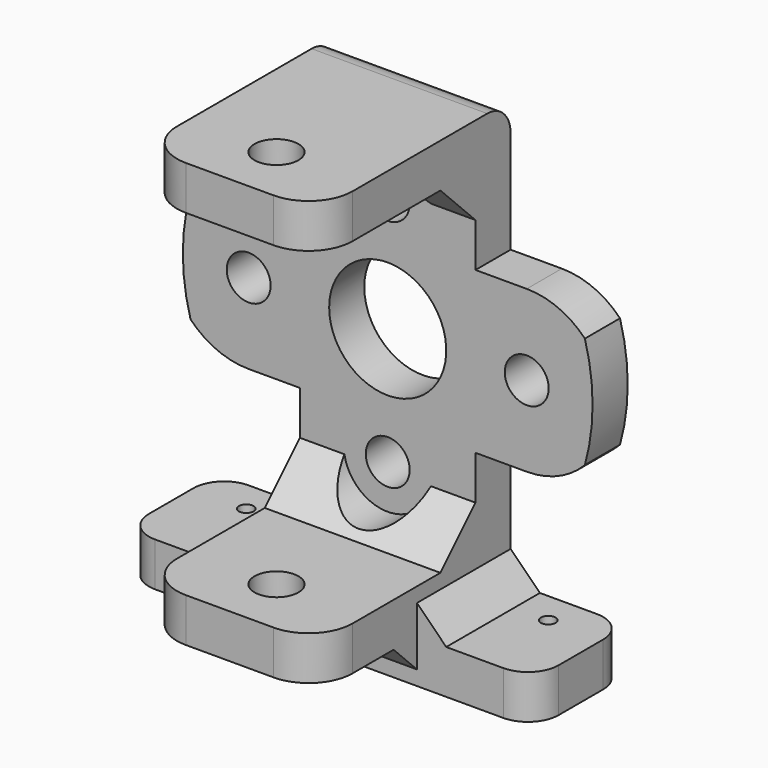
from build123d import *

# Parameters (mm, degrees)
F0_R          = 1.5
F0_R_2        = 4.5
F1_DEPTH      = 3
F2_W          = 12
F2_H          = 29
F3_DEPTH      = 3
F4_R          = 1.5
F5_DEPTH      = 3
F6_R          = 4
F6_R_2        = 1.5
F7_DEPTH      = 3
F9_R          = 2
F10_T4_DEPTH  = 12
F10_S5_R      = 1.5
F10_T6_DEPTH  = 8
F10_T10_DEPTH = 12
F10_S11_R     = 1.5
F10_T12_DEPTH = 8
F11_R         = 3
F12_DEPTH     = 4
F13_R         = 0.5
F14_DEPTH     = 3
F15_T1_DEPTH  = 8
F16_T1_DEPTH  = 8
F17_SIZE      = 2


# Not quite as in the source:
# - a fillet or chamfer that OpenCascade refuses, or shapes differently, is made with other operations: its cross-section is extruded or revolved along the edge and cut away or added


with BuildPart() as f1:
    # F0 (on Front) → F1 (new body)
    with BuildSketch(Plane.XZ):
        with BuildLine():
            Line((0, -5.5), (9.5, -5.5))
            ThreePointArc((9.5, -5.5), (11.6605151609, -5.0578823869), (13.4736842105, -3.8026088144))
            ThreePointArc((13.4736842105, -3.8026088144), (14, 0), (13.4736842105, 3.8026088144))
            ThreePointArc((13.4736842105, 3.8026088144), (11.6605151609, 5.0578823869), (9.5, 5.5))
            Line((9.5, 5.5), (0, 5.5))
            Line((0, 5.5), (-9.5, 5.5))
            ThreePointArc((-9.5, 5.5), (-11.6605151609, 5.0578823869), (-13.4736842105, 3.8026088144))
            ThreePointArc((-13.4736842105, 3.8026088144), (-14, 0), (-13.4736842105, -3.8026088144))
            ThreePointArc((-13.4736842105, -3.8026088144), (-11.6605151609, -5.0578823869), (-9.5, -5.5))
            Line((-9.5, -5.5), (0, -5.5))
        make_face()
        with Locations((-9.5, 0)):
            Circle(F0_R, mode=Mode.SUBTRACT)
        Circle(F0_R_2, mode=Mode.SUBTRACT)
        with Locations((9.5, 0)):
            Circle(F0_R, mode=Mode.SUBTRACT)
    extrude(amount=F1_DEPTH)

    # F2 (on face) → F3 (join)
    with BuildSketch(Plane.XZ.offset(3)):
        Rectangle(F2_W, F2_H)
    extrude(amount=-F3_DEPTH)

    # F4 (on face) → F5 (join)
    with BuildSketch(Plane(origin=(0, 0, -14.5), x_dir=(1, 0, 0), z_dir=(0, 0, -1))):
        with BuildLine():
            Line((-6, 13.5), (-6, 0))
            Line((-6, 0), (6, 0))
            Line((6, 0), (6, 13.5))
            ThreePointArc((6, 13.5), (5.1213203436, 15.6213203436), (3, 16.5))
            Line((3, 16.5), (-3, 16.5))
            ThreePointArc((-3, 16.5), (-5.1213203436, 15.6213203436), (-6, 13.5))
        make_face()
        with Locations((0, 12.5)):
            Circle(F4_R, mode=Mode.SUBTRACT)
    extrude(amount=-F5_DEPTH)

    # F6 (on face) → F7 (cut, through all)
    with BuildSketch(Plane(origin=(0, 0, 0), x_dir=(-1, 0, 0), z_dir=(0, 1, 0))):
        Circle(F6_R)
        with Locations((0, 8)):
            Circle(F6_R_2)
        with Locations((0, -8)):
            Circle(F6_R_2)
    extrude(amount=-F7_DEPTH, mode=Mode.SUBTRACT)

    # F8: F1 across plane


with BuildPart() as f1_1:
    add(f1.part)
    add(f1.part.mirror(Plane.XY))

    # F9
    f9_edges = [f1_1.edges().sort_by_distance(p)[0] for p in [
        (0, 0, 14.5),
    ]]
    fillet(f9_edges, radius=F9_R)

    # F10: chamfer of 3 on 2 edges, made by hand


with BuildPart() as f10_tool2:
    # F10_s3 → F10_t4 (new body)
    with BuildSketch(Plane.YZ.offset(-6)):
        Polygon((-3, 8.5), (-6, 11.5), (-3, 11.5), align=None)
    extrude(amount=F10_T4_DEPTH)

    # F10_s5 → F10_t6 (cut, symmetric)
    with BuildSketch(Plane.XZ.offset(4.5)):
        with Locations((0, 8)):
            Circle(F10_S5_R)
    extrude(amount=F10_T6_DEPTH, both=True, mode=Mode.SUBTRACT)


with BuildPart() as f1_2:
    add(f1_1.part)

    # F10_t1: union F10_tool2
    add(f10_tool2.part)


with BuildPart() as f10_tool8:
    # F10_s9 → F10_t10 (new body)
    with BuildSketch(Plane.YZ.offset(-6)):
        Polygon((-3, -8.5), (-6, -11.5), (-3, -11.5), align=None)
    extrude(amount=F10_T10_DEPTH)

    # F10_s11 → F10_t12 (cut, symmetric)
    with BuildSketch(Plane.XZ.offset(4.5)):
        with Locations((0, -8)):
            Circle(F10_S11_R)
    extrude(amount=F10_T12_DEPTH, both=True, mode=Mode.SUBTRACT)


with BuildPart() as f1_3:
    add(f1_2.part)

    # F10_t7: union F10_tool8
    add(f10_tool8.part)

    # F11 (on face) → F12 (cut)
    with BuildSketch(Plane.XZ.offset(3)):
        with Locations((0, 8)):
            Circle(F11_R)
        with Locations((0, -8)):
            Circle(F11_R)
    extrude(amount=F12_DEPTH, mode=Mode.SUBTRACT)

    # F13 (on face) → F14 (join)
    with BuildSketch(Plane(origin=(0, 0, -14.5), x_dir=(1, 0, 0), z_dir=(0, 0, -1))):
        with BuildLine():
            Line((-11.9, 0), (6, 0))
            Line((6, 0), (6, 8))
            Line((6, 8), (-11.9, 8))
            ThreePointArc((-11.9, 8), (-13.3849242405, 7.3849242405), (-14, 5.9))
            Line((-14, 5.9), (-14, 2.1))
            ThreePointArc((-14, 2.1), (-13.3849242405, 0.6150757595), (-11.9, 0))
        make_face()
        with Locations((-10.3164756671, 2.1835243329)):
            Circle(F13_R, mode=Mode.SUBTRACT)
        with BuildLine():
            Line((6, 8), (6, 0))
            Line((6, 0), (11.9, 0))
            ThreePointArc((11.9, 0), (13.3849242405, 0.6150757595), (14, 2.1))
            Line((14, 2.1), (14, 5.9))
            ThreePointArc((14, 5.9), (13.3849242405, 7.3849242405), (11.9, 8))
            Line((11.9, 8), (6, 8))
        make_face()
        with Locations((10.3164756671, 2.1835243329)):
            Circle(F13_R, mode=Mode.SUBTRACT)
    extrude(amount=F14_DEPTH)

    # F15: chamfer of 2 on 1 edges, made by hand

    # F15_s2 → F15_t1 (join)
    with BuildSketch(Plane.XZ):
        Polygon((-6, -12.5), (-8, -14.5), (-6, -14.5), align=None)
    extrude(amount=F15_T1_DEPTH)

    # F16: chamfer of 2 on 1 edges, made by hand

    # F16_s2 → F16_t1 (join)
    with BuildSketch(Plane.XZ):
        Polygon((8, -14.5), (6, -12.5), (6, -14.5), align=None)
    extrude(amount=F16_T1_DEPTH)

    # F17
    f17_edges = [f1_3.edges().sort_by_distance(p)[0] for p in [
        (0, -8, -14.5),
    ]]
    chamfer(f17_edges, length=F17_SIZE)


solid = f1_3.part
